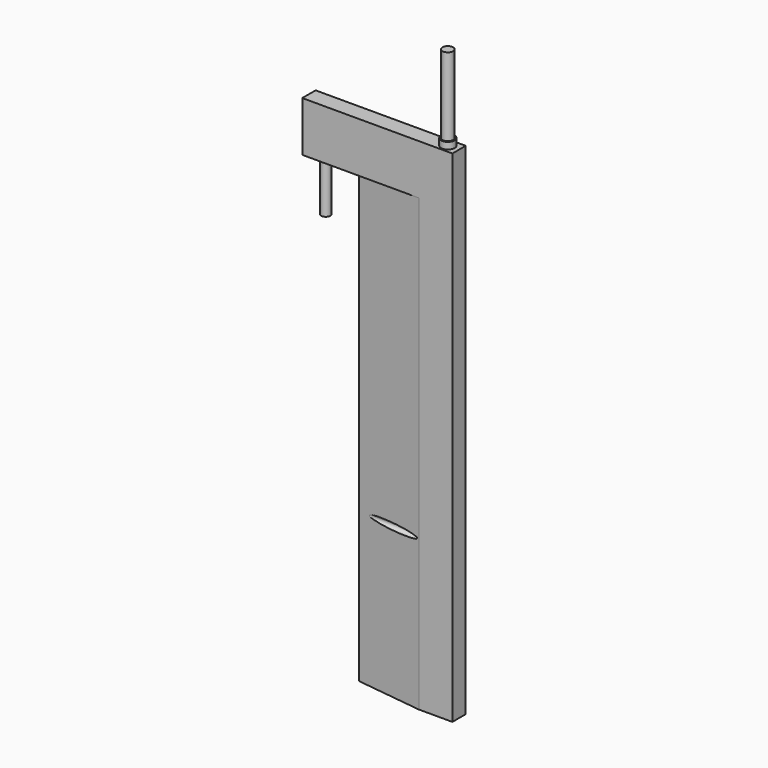
from build123d import *

# Parameters (mm, degrees)
F0_W      = 30
F0_H      = 150
F1_DEPTH  = 5
F3_DEPTH  = 150.001
F2_R      = 1.5989652731
F4_DEPTH  = 140
F5_R      = 1
F6_DEPTH  = 25.5216695368
F7_DEPTH  = 15
F9_DEPTH  = 15
F10_R     = 1.4
F11_DEPTH = 30
F13_DEPTH = 25.4
F12_R     = 2.0390969853
F14_DEPTH = 2


with BuildPart() as f1:
    # F0 (on Front) → F1 (new body)
    with BuildSketch(Plane.XZ):
        with Locations((15, -75)):
            Rectangle(F0_W, F0_H)
    extrude(amount=F1_DEPTH)

    # F2 (on face) → F3 (cut, through all)
    with BuildSketch(Plane.XY):
        Polygon((0, -2.5), (19.9251845479, 0), (0, 0), align=None)
        Polygon((19.9251845479, -5), (0, -2.5), (0, -5), align=None)
    extrude(amount=-F3_DEPTH, mode=Mode.SUBTRACT)

    # F2 (on face) → F4 (cut)
    with BuildSketch(Plane.XY):
        with Locations((26.6364086419, -2.5)):
            Circle(F2_R)
    extrude(amount=-F4_DEPTH, mode=Mode.SUBTRACT)

    # F5 (on Right) → F6 (cut)
    with BuildSketch(Plane.YZ):
        with Locations((-3.9339680225, -104.9845516682)):
            Circle(F5_R)
    extrude(amount=F6_DEPTH, mode=Mode.SUBTRACT)

    # F2 (on face) → F7 (join)
    with BuildSketch(Plane.XY):
        Polygon((0, -2.5), (19.9251845479, 0), (0, 0), align=None)
        Polygon((30, 0), (19.9251845479, 0), (0, -2.5), (19.9251845479, -5), (30, -5), align=None)
        with Locations((26.6364086419, -2.5)):
            Circle(F2_R, mode=Mode.SUBTRACT)
        Polygon((19.9251845479, -5), (0, -2.5), (0, -5), align=None)
    extrude(amount=-F7_DEPTH)

    # F8 (on face) → F9 (join)
    with BuildSketch(Plane(origin=(0, 0, 0), x_dir=(0, -1, 0), z_dir=(-1, 0, 0))):
        Polygon((5, 0), (0, 0), (0, -15), (2.5, -15), (5, -15), align=None)
    extrude(amount=F9_DEPTH)

    # F10 (on face) → F11 (join)
    with BuildSketch(Plane.XY):
        with Locations((-9.9609950557, -2.5)):
            Circle(F10_R)
    extrude(amount=-F11_DEPTH)


with BuildPart() as f13:
    # F2 (on face) → F13 (new body)
    with BuildSketch(Plane.XY):
        with Locations((26.6364086419, -2.5)):
            Circle(F2_R)
    extrude(amount=F13_DEPTH)


with BuildPart() as f14:
    # F12 (on face) → F14 (new body)
    with BuildSketch(Plane.XY):
        with Locations((26.6568399966, -2.5064747315)):
            Circle(F12_R)
        with BuildLine():
            ThreePointArc((26.4101542038, -0.9171232285), (27.7032928469, -1.2850704117), (28.2652218171, -2.5064747315))
            ThreePointArc((28.2652218171, -2.5064747315), (27.2854196118, -3.9869407891), (25.5397747623, -3.6636511842))
            ThreePointArc((25.5397747623, -3.6636511842), (25.112150682, -2.0169600262), (26.4101542038, -0.9171232285))
        make_face(mode=Mode.SUBTRACT)
    extrude(amount=F14_DEPTH)


solid = Compound([f1.part, f13.part, f14.part])
